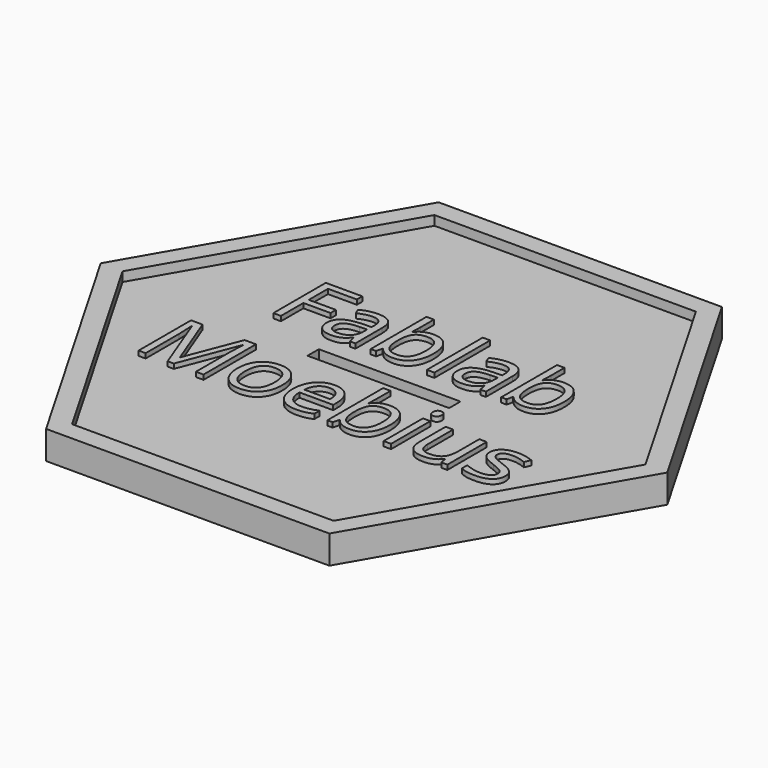
from build123d import *

# Parameters (mm, degrees)
F0_W         = 30
F0_H         = 3
F1_DEPTH     = 6
F3_DEPTH     = 2
F4_W         = 30
F4_H         = 3
F5_DEPTH     = 2
F6_TEXT_SIZE = 19.4444444444
F7_DEPTH     = 1


# Not quite as in the source:
# - Text() gives the source's letters only with a copy of the font that has no kerning and outlines rounded to 1/6400 em; it was checked with that copy


with BuildPart() as f1:
    # F0 (on Top) → F1 (new body)
    with BuildSketch(Plane.XY):
        Polygon((30, -51.9615242271), (60, 0), (30, 51.9615242271), (-30, 51.9615242271), (-60, 0), (-30, -51.9615242271), align=None)
        Rectangle(F0_W, F0_H, mode=Mode.SUBTRACT)
    extrude(amount=F1_DEPTH)

    # F2 (on face) → F3 (cut)
    with BuildSketch(Plane(origin=(0, 0, 0), x_dir=(1, 0, 0), z_dir=(0, 0, -1))):
        Polygon((-27.6905989232, -47.9615242271), (27.6905989232, -47.9615242271), (55.3811978465, 0), (27.6905989232, 47.9615242271), (-27.6905989232, 47.9615242271), (-55.3811978465, 0), align=None)
        Polygon((51.9170962313, 0), (25.9585481157, -44.9615242271), (-25.9585481157, -44.9615242271), (-51.9170962313, 0), (-25.9585481157, 44.9615242271), (25.9585481157, 44.9615242271), align=None, mode=Mode.SUBTRACT)
    extrude(amount=-F3_DEPTH, mode=Mode.SUBTRACT)

    # F4 (on face) → F5 (cut)
    with BuildSketch(Plane.XY.offset(6)):
        Polygon((-55.3811978465, 0), (-27.6905989232, -47.9615242271), (27.6905989232, -47.9615242271), (55.3811978465, 0), (27.6905989232, 47.9615242271), (-27.6905989232, 47.9615242271), align=None)
        Rectangle(F4_W, F4_H, mode=Mode.SUBTRACT)
    extrude(amount=-F5_DEPTH, mode=Mode.SUBTRACT)

    # F6 (on face) → F7 (join)
    with BuildSketch(Plane.XY.offset(4)):
        with Locations((-38.6807725694, -19)):
            Text('Moebius', F6_TEXT_SIZE, font='Open Sans', text_align=(TextAlign.LEFT, TextAlign.BOTTOM))
        with Locations((-29.6649305556, 5.3990301341)):
            Text('Fablab', F6_TEXT_SIZE, font='Open Sans', text_align=(TextAlign.LEFT, TextAlign.BOTTOM))
    extrude(amount=F7_DEPTH)


solid = f1.part
